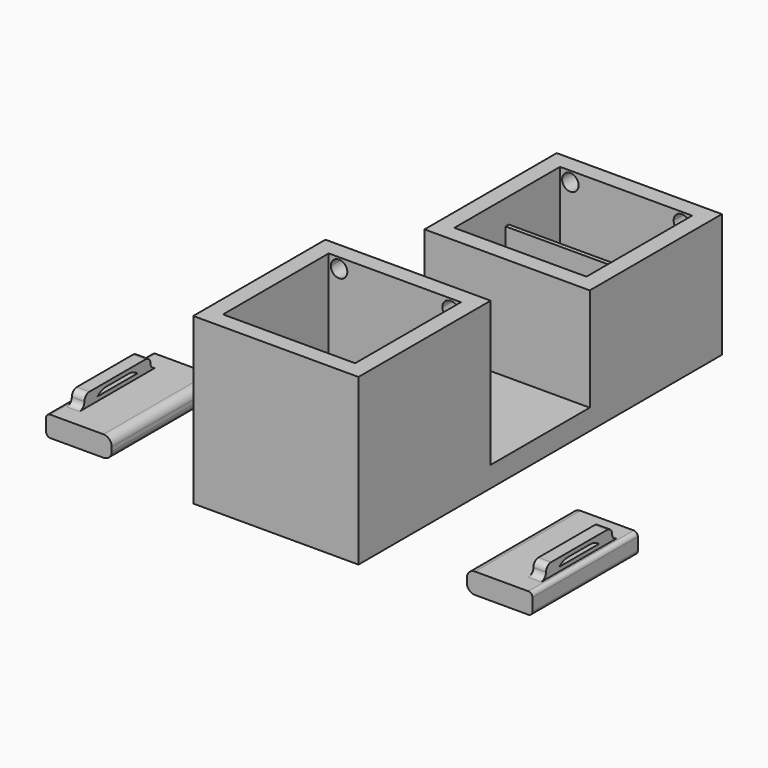
from build123d import *

# Parameters (mm, degrees)
F0_W         = 50.8
F0_H         = 50.8
F1_DEPTH     = 50.8
F2_DEPTH     = 38.1
F0_H_2       = 38.1
F3_DEPTH     = 6.35
F4_T         = -5.08
F6_DEPTH     = 50.8
F7_W         = 20.193
F7_H         = 40.513
F8_DEPTH     = 6.35
F11_DEPTH    = 3.81
F12_W        = 7.62
F12_H        = 1.27
F13_DEPTH    = 25.4
F14_R        = 1.90499
F15_T1_DEPTH = 3.8801973377
F16_R        = 2.54
F17_DEPTH    = 50.8
F18_R        = 2.54
F19_R        = 1.27
F20_W        = 40.64
F20_H        = 0.635
F21_DEPTH    = 25.4
F22_DEPTH    = 25.4


# Not quite as in the source:
# - a fillet or chamfer that OpenCascade refuses, or shapes differently, is made with other operations: its cross-section is extruded or revolved along the edge and cut away or added
# - a fillet or chamfer is up to 0.001 mm smaller than in the source, because OpenCascade refuses the exact size


with BuildPart() as f1:
    # F0 (on Top) → F1 (new body)
    with BuildSketch(Plane.XY):
        Rectangle(F0_W, F0_H)
    extrude(amount=F1_DEPTH)



with BuildPart() as f2:
    # F0 (on Top) → F2 (new body)
    with BuildSketch(Plane.XY):
        with Locations((0, 88.9)):
            Rectangle(F0_W, F0_H)
    extrude(amount=F2_DEPTH)


with BuildPart() as f1_1:
    add(f1.part)

    add(f2.part)  # F3 merges F2
    # F0 (on Top) → F3 (join)
    with BuildSketch(Plane.XY):
        with Locations((0, 44.45)):
            Rectangle(F0_W, F0_H_2)
    extrude(amount=F3_DEPTH)

    # F4
    f4_openings = [f1_1.faces().sort_by_distance(p)[0] for p in [
        (0, 88.9, 38.1),
        (0, 0, 50.8),
    ]]
    offset(amount=F4_T, openings=f4_openings, kind=Kind.INTERSECTION)

    # F5 (on face) → F6 (cut)
    with BuildSketch(Plane(origin=(0, -20.32, 0), x_dir=(-1, 0, 0), z_dir=(0, 1, 0))):
        with BuildLine():
            ThreePointArc((-17.145, 50.165), (-18.9410512242, 45.8289487758), (-14.605, 47.625))
            ThreePointArc((-14.605, 47.625), (-15.3489487758, 49.4210512242), (-17.145, 50.165))
        make_face()
        with BuildLine():
            ThreePointArc((17.145, 50.165), (15.3489487758, 45.8289487758), (19.685, 47.625))
            ThreePointArc((19.685, 47.625), (18.9410512242, 49.4210512242), (17.145, 50.165))
        make_face()
    extrude(amount=F6_DEPTH, mode=Mode.SUBTRACT)

    # F16 (on face) → F17 (cut)
    with BuildSketch(Plane(origin=(0, 68.58, 0), x_dir=(-1, 0, 0), z_dir=(0, 1, 0))):
        with BuildLine():
            ThreePointArc((-14.605, 34.925), (-15.3489487758, 36.7210512242), (-17.145, 37.465))
            ThreePointArc((-17.145, 37.465), (-18.9410512242, 33.1289487758), (-14.605, 34.925))
        make_face()
        with Locations((17.145, 34.925)):
            Circle(F16_R)
    extrude(amount=F17_DEPTH, mode=Mode.SUBTRACT)

    # F20 (on face) → F21 (join)
    with BuildSketch(Plane.XY.offset(5.08)):
        with Locations((0, 89.2175)):
            Rectangle(F20_W, F20_H)
        with Locations((0, 88.5825)):
            Rectangle(F20_W, F20_H)
    extrude(amount=F21_DEPTH)


with BuildPart() as f8:
    # F7 (on Top) → F8 (new body)
    with BuildSketch(Plane.XY):
        with Locations((-64.6820784919, 0)):
            Rectangle(F7_W, F7_H)
    extrude(amount=F8_DEPTH)

    # F10 (on face) → F11 (join)
    with BuildSketch(Plane.XY.offset(6.35)):
        Polygon((-72.9086771607, 12.7), (-72.9086771607, 0), (-72.9086771607, -12.7), (-69.028479823, -12.7), (-69.028479823, 12.7), align=None)
    extrude(amount=F11_DEPTH)

    # F12 (on face) → F13 (cut)
    with BuildSketch(Plane(origin=(-72.9086771607, 0, 0), x_dir=(0, -1, 0), z_dir=(-1, 0, 0))):
        with Locations((-3.81, 8.255)):
            Rectangle(F12_W, F12_H)
        with Locations((3.81, 8.255)):
            Rectangle(F12_W, F12_H)
    extrude(amount=-F13_DEPTH, mode=Mode.SUBTRACT)

    # F14 (radius 1.905 in the source; OpenCascade refuses exactly that, so slightly less here)
    f14_edges = [f8.edges().sort_by_distance(p)[0] for p in [
        (-70.968578, -12.7, 10.16),
        (-70.968578, 12.7, 10.16),
        (-70.968578, 12.7, 6.35),
        (-70.968578, -12.7, 6.35),
    ]]
    fillet(f14_edges, radius=F14_R)

    # F15: fillet of radius 5.08 on 2 edges, made by hand

    # F15_s2 → F15_t1 (join)
    with BuildSketch(Plane.YZ.offset(-72.9086771607)):
        with BuildLine():
            ThreePointArc((-7.62, 7.62), (-6.0559470592, 8.5619048812), (-4.2598958349, 8.89))
            Line((-4.2598958349, 8.89), (-7.62, 8.89))
            Line((-7.62, 8.89), (-7.62, 7.62))
        make_face()
        with BuildLine():
            ThreePointArc((4.2598958349, 8.89), (6.0559470592, 8.5619048812), (7.62, 7.62))
            Line((7.62, 7.62), (7.62, 8.89))
            Line((7.62, 8.89), (4.2598958349, 8.89))
        make_face()
    extrude(amount=F15_T1_DEPTH)

    # F18
    f18_edges = [f8.edges().sort_by_distance(p)[0] for p in [
        (-54.585578, 0, 6.35),
        (-54.585578, 0, 0),
    ]]
    fillet(f18_edges, radius=F18_R)

    # F19
    f19_edges = [f8.edges().sort_by_distance(p)[0] for p in [
        (-74.778578, 0, 6.35),
        (-74.778578, 0, 0),
    ]]
    fillet(f19_edges, radius=F19_R)

    # F9 (on face) → F22 (cut)
    with BuildSketch(Plane(origin=(0, 20.2565, 0), x_dir=(-1, 0, 0), z_dir=(0, 1, 0))):
        with BuildLine():
            ThreePointArc((60.3005784919, 3.175), (57.7605784919, 5.715), (55.2205784919, 3.175))
            ThreePointArc((55.2205784919, 3.175), (57.7605784919, 0.635), (60.3005784919, 3.175))
        make_face()
    extrude(amount=-F22_DEPTH, mode=Mode.SUBTRACT)


with BuildPart() as f23_1:
    # F23: instance of F8
    add(f8.part.mirror(Plane.YZ))


solid = Compound([f1_1.part, f8.part, f23_1.part])
